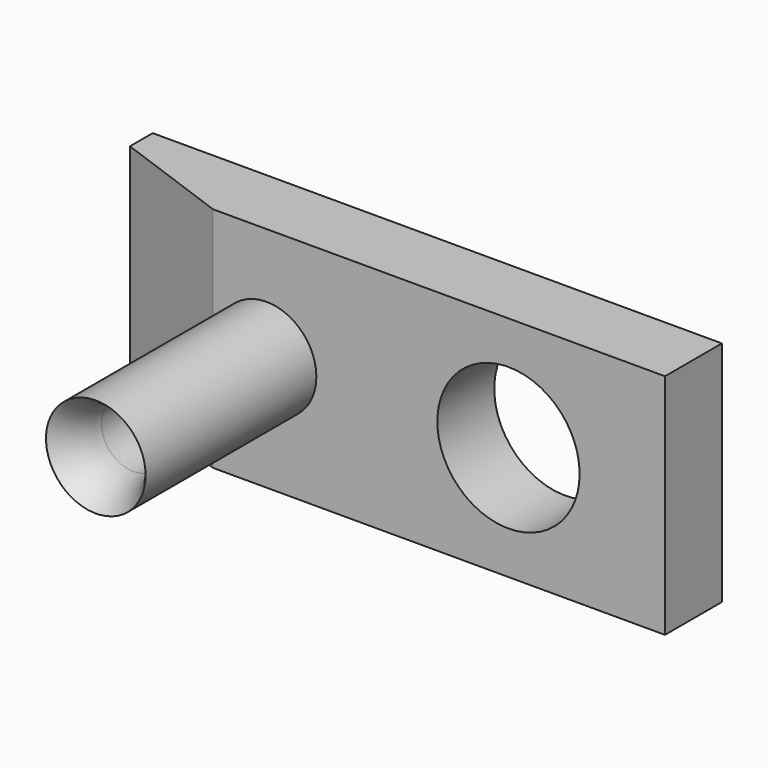
from build123d import *

# Parameters (mm, degrees)
F0_R     = 5
F1_DEPTH = 5
F2_R     = 3.5
F2_R_2   = 2.25
F3_DEPTH = 15
F5_SIZE2 = 8.2424322584
F5_SIZE  = 3


# Not quite as in the source:
# - a fillet or chamfer that OpenCascade refuses, or shapes differently, is made with other operations: its cross-section is extruded or revolved along the edge and cut away or added


with BuildPart() as f1:
    # F0 (on Front) → F1 (new body)
    with BuildSketch(Plane.XZ):
        Polygon((-20, -8), (20, -8), (20, 0), (20, 8), (-20, 8), (-20, 0), align=None)
        with BuildLine():
            ThreePointArc((-6, 0), (-8, -2), (-10, 0))
            ThreePointArc((-10, 0), (-8, 2), (-6, 0))
        make_face(mode=Mode.SUBTRACT)
        with Locations((9, 0)):
            Circle(F0_R, mode=Mode.SUBTRACT)
    extrude(amount=F1_DEPTH)

    # F2 (on face) → F3 (join)
    with BuildSketch(Plane.XZ.offset(5)):
        with Locations((-8, 0)):
            Circle(F2_R)
        with Locations((-8, 0)):
            Circle(F2_R_2, mode=Mode.SUBTRACT)
    extrude(amount=F3_DEPTH)

    # F4: fillet of radius 5 on 1 edges, made by hand

    # F4_s1 → F4_t2 (revolve, cut)
    with BuildSketch(Plane.XY):
        with BuildLine():
            ThreePointArc((-4.5, -20), (-5.4270717335, -18.4605778141), (-5.75, -16.6928108612))
            Line((-5.75, -16.6928108612), (-5.75, -20))
            Line((-5.75, -20), (-4.5, -20))
        make_face()
    revolve(axis=Axis((-8, -20, 0), (0, -1, 0)), mode=Mode.SUBTRACT)

    # F5
    f5_edges = [f1.edges().sort_by_distance(p)[0] for p in [
        (-20, -5, 0),
    ]]
    f5_side = f1.faces().sort_by_distance((-20, -2.5, 0))[0]
    chamfer(f5_edges, length=F5_SIZE, length2=F5_SIZE2, reference=f5_side)


solid = f1.part
